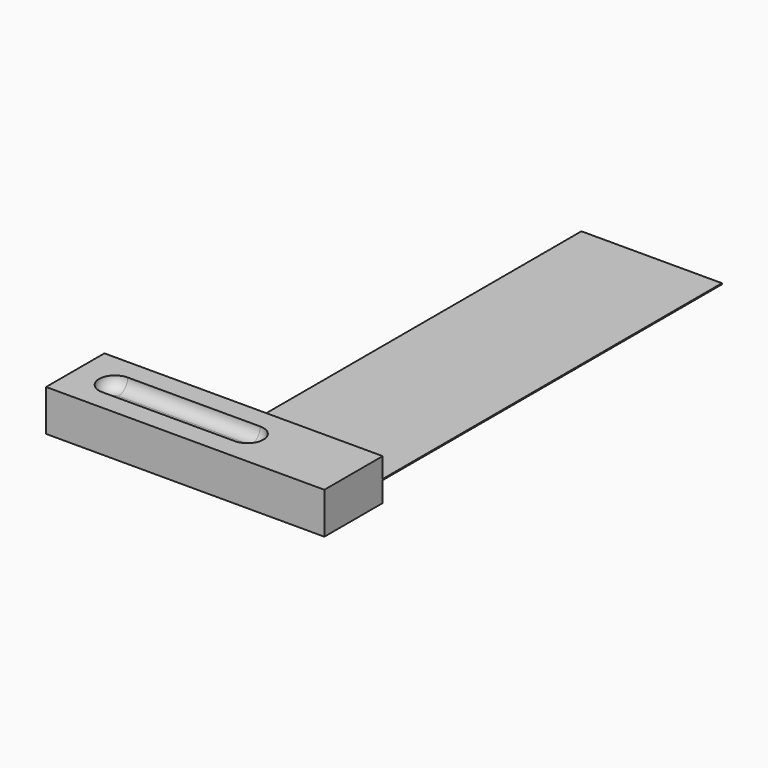
from build123d import *

# Parameters (mm, degrees)
F0_W     = 133.35
F0_H     = 34.925
F1_DEPTH = 19.812
F3_DEPTH = 5.588
F5_DEPTH = 203.2
F6_R     = 5.58799


# Not quite as in the source:
# - a fillet or chamfer is up to 0.001 mm smaller than in the source, because OpenCascade refuses the exact size


with BuildPart() as f1:
    # F0 (on Top) → F1 (new body)
    with BuildSketch(Plane.XY):
        with Locations((0.6578612807, 43.2195533067)):
            Rectangle(F0_W, F0_H)
    extrude(amount=F1_DEPTH)

    # F2 (on face) → F3 (cut)
    with BuildSketch(Plane.XY.offset(19.812)):
        with BuildLine():
            ThreePointArc((16.5328612807, 35.600391914), (24.1524419771, 43.2199726103), (16.5328612807, 50.8395533067))
            Line((16.5328612807, 50.8395533067), (-46.9671387193, 50.8395533067))
            ThreePointArc((-46.9671387193, 50.8395533067), (-54.5869290646, 43.276078466), (-47.0801859275, 35.600391914))
            Line((-47.0801859275, 35.600391914), (16.5328612807, 35.600391914))
        make_face()
    extrude(amount=-F3_DEPTH, mode=Mode.SUBTRACT)

    # F6 (radius 5.588 in the source; OpenCascade refuses exactly that, so slightly less here)
    f6_edges = [f1.edges().sort_by_distance(p)[0] for p in [
        (24.152442, 43.219973, 14.224),
        (-15.217139, 50.839553, 14.224),
        (-54.586929, 43.276078, 14.224),
        (-15.273662, 35.600392, 14.224),
    ]]
    fillet(f6_edges, radius=F6_R)


with BuildPart() as f5:
    # F4 (on face) → F5 (new body)
    with BuildSketch(Plane(origin=(0, 60.6820533067, 0), x_dir=(-1, 0, 0), z_dir=(0, 1, 0))):
        Polygon((0, 9.6509261072), (0, 9.906), (0, 10.1556647569), (0, 10.1610738928), (-67.3328612807, 10.1610738928), (-67.3328612807, 9.6509261072), align=None)
    extrude(amount=F5_DEPTH)


solid = Compound([f1.part, f5.part])
